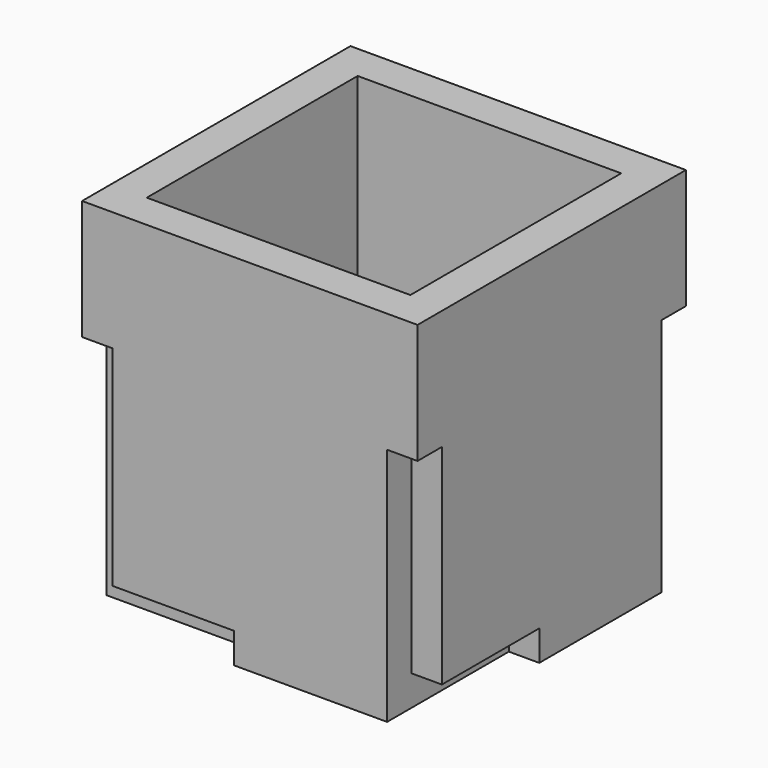
from build123d import *

# Parameters (mm, degrees)
F0_W     = 440
F0_H     = 440
F1_DEPTH = 50.8
F0_W_2   = 50.8
F0_H_2   = 203.2
F0_W_3   = 203.2
F0_H_3   = 50.8
F2_DEPTH = 349.2
F3_DEPTH = 149.2
F4_W     = 440
F4_H     = 440
F4_W_2   = 50.8
F4_H_2   = 50.8
F5_DEPTH = 200


# Not quite as in the source:
# - a feature names something its author has since deleted; it is built from what else it names


with BuildPart() as f1:
    # F0 (on Top) → F1 (new body)
    with BuildSketch(Plane.XY):
        Polygon((91.7435496044, 289.8852448295), (-163.4564503956, 289.8852448295), (-163.4564503956, 239.0852448295), (-163.4564503956, 35.8852448295), (-214.2564503956, 35.8852448295), (-214.2564503956, -219.3147551705), (-163.4564503956, -219.3147551705), (39.7435496044, -219.3147551705), (39.7435496044, -270.1147551705), (294.9435496044, -270.1147551705), (294.9435496044, -219.3147551705), (294.9435496044, -16.1147551705), (345.7435496044, -16.1147551705), (345.7435496044, 239.0852448295), (294.9435496044, 239.0852448295), (91.7435496044, 239.0852448295), align=None)
        with Locations((65.7435496044, 9.8852448295)):
            Rectangle(F0_W, F0_H, mode=Mode.SUBTRACT)
        with Locations((65.7435496044, 9.8852448295)):
            Rectangle(F0_W, F0_H)
        Polygon((-65.0564503956, 140.6852448295), (-14.2564503956, 140.6852448295), (87.3435496044, 140.6852448295), (196.5435496044, 140.6852448295), (196.5435496044, 89.8852448295), (196.5435496044, -11.7147551705), (196.5435496044, -120.9147551705), (145.7435496044, -120.9147551705), (44.1435496044, -120.9147551705), (-65.0564503956, -120.9147551705), (-65.0564503956, -70.1147551705), (-65.0564503956, 31.4852448295), align=None, mode=Mode.SUBTRACT)
        Polygon((87.3435496044, 89.8852448295), (-14.2564503956, 89.8852448295), (-14.2564503956, 140.6852448295), (-65.0564503956, 140.6852448295), (-65.0564503956, 31.4852448295), (-14.2564503956, 31.4852448295), (-14.2564503956, -70.1147551705), (-65.0564503956, -70.1147551705), (-65.0564503956, -120.9147551705), (44.1435496044, -120.9147551705), (44.1435496044, -70.1147551705), (145.7435496044, -70.1147551705), (145.7435496044, -120.9147551705), (196.5435496044, -120.9147551705), (196.5435496044, -11.7147551705), (145.7435496044, -11.7147551705), (145.7435496044, 89.8852448295), (196.5435496044, 89.8852448295), (196.5435496044, 140.6852448295), (87.3435496044, 140.6852448295), align=None)
    extrude(amount=-F1_DEPTH)

    # F0 (on Top) → F2 (join)
    with BuildSketch(Plane.XY):
        Polygon((91.7435496044, 289.8852448295), (-163.4564503956, 289.8852448295), (-163.4564503956, 239.0852448295), (-163.4564503956, 35.8852448295), (-214.2564503956, 35.8852448295), (-214.2564503956, -219.3147551705), (-163.4564503956, -219.3147551705), (39.7435496044, -219.3147551705), (39.7435496044, -270.1147551705), (294.9435496044, -270.1147551705), (294.9435496044, -219.3147551705), (294.9435496044, -16.1147551705), (345.7435496044, -16.1147551705), (345.7435496044, 239.0852448295), (294.9435496044, 239.0852448295), (91.7435496044, 239.0852448295), align=None)
        with Locations((65.7435496044, 9.8852448295)):
            Rectangle(F0_W, F0_H, mode=Mode.SUBTRACT)
        with Locations((320.3435496044, -117.7147551705)):
            Rectangle(F0_W_2, F0_H_2)
        with Locations((193.3435496044, 264.4852448295)):
            Rectangle(F0_W_3, F0_H_3)
        with Locations((-188.8564503956, 137.4852448295)):
            Rectangle(F0_W_2, F0_H_2)
        with Locations((-61.8564503956, -244.7147551705)):
            Rectangle(F0_W_3, F0_H_3)
    extrude(amount=F2_DEPTH)

    # F0 (on Top) → F3 (join)
    with BuildSketch(Plane.XY):
        with Locations((65.7435496044, 9.8852448295)):
            Rectangle(F0_W, F0_H)
        Polygon((-65.0564503956, 140.6852448295), (-14.2564503956, 140.6852448295), (87.3435496044, 140.6852448295), (196.5435496044, 140.6852448295), (196.5435496044, 89.8852448295), (196.5435496044, -11.7147551705), (196.5435496044, -120.9147551705), (145.7435496044, -120.9147551705), (44.1435496044, -120.9147551705), (-65.0564503956, -120.9147551705), (-65.0564503956, -70.1147551705), (-65.0564503956, 31.4852448295), align=None, mode=Mode.SUBTRACT)
        Polygon((87.3435496044, 89.8852448295), (-14.2564503956, 89.8852448295), (-14.2564503956, 140.6852448295), (-65.0564503956, 140.6852448295), (-65.0564503956, 31.4852448295), (-14.2564503956, 31.4852448295), (-14.2564503956, -70.1147551705), (-65.0564503956, -70.1147551705), (-65.0564503956, -120.9147551705), (44.1435496044, -120.9147551705), (44.1435496044, -70.1147551705), (145.7435496044, -70.1147551705), (145.7435496044, -120.9147551705), (196.5435496044, -120.9147551705), (196.5435496044, -11.7147551705), (145.7435496044, -11.7147551705), (145.7435496044, 89.8852448295), (196.5435496044, 89.8852448295), (196.5435496044, 140.6852448295), (87.3435496044, 140.6852448295), align=None)
    extrude(amount=F3_DEPTH)

    # F4 (on face) → F5 (join)
    with BuildSketch(Plane.XY.offset(349.2)):
        Polygon((-163.4564503956, -219.3147551705), (-163.4564503956, -270.1147551705), (294.9435496044, -270.1147551705), (294.9435496044, -219.3147551705), (345.7435496044, -219.3147551705), (345.7435496044, 239.0852448295), (294.9435496044, 239.0852448295), (294.9435496044, 289.8852448295), (-163.4564503956, 289.8852448295), (-163.4564503956, 239.0852448295), (-214.2564503956, 239.0852448295), (-214.2564503956, -219.3147551705), align=None)
        with Locations((65.7435496044, 9.8852448295)):
            Rectangle(F4_W, F4_H, mode=Mode.SUBTRACT)
        with Locations((-188.8564503956, -244.7147551705)):
            Rectangle(F4_W_2, F4_H_2)
        with Locations((320.3435496044, 264.4852448295)):
            Rectangle(F4_W_2, F4_H_2)
        with Locations((-188.8564503956, 264.4852448295)):
            Rectangle(F4_W_2, F4_H_2)
        with Locations((320.3435496044, -244.7147551705)):
            Rectangle(F4_W_2, F4_H_2)
    extrude(amount=F5_DEPTH)


solid = f1.part
